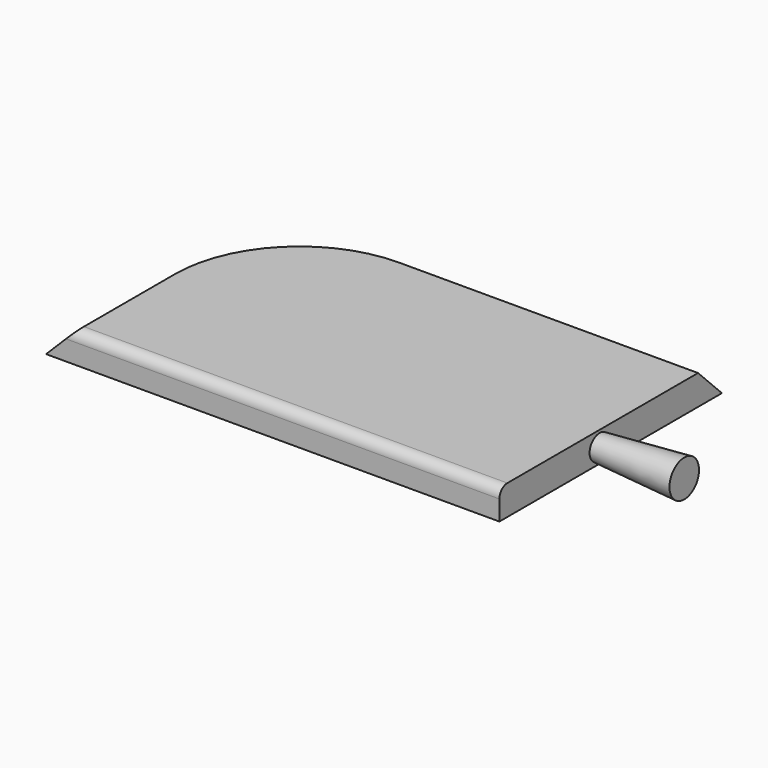
from build123d import *

# Parameters (mm, degrees)
F1_DEPTH    = 15.24
F2_T1_DEPTH = 217.8918149653
F2_T3_DEPTH = 128.5071697417
F2_T6_ANGLE = 90
F3_R        = 5.08
F4_R        = 6.3991299939
F5_DEPTH    = 43.18
F5_TAPER    = -4


# Not quite as in the source:
# - a fillet or chamfer that OpenCascade refuses, or shapes differently, is made with other operations: its cross-section is extruded or revolved along the edge and cut away or added


with BuildPart() as f1:
    # F0 (on Top) → F1 (new body)
    with BuildSketch(Plane.XY):
        with BuildLine():
            Line((120.7355335355, 76.0432109237), (-31.8355335355, 76.0432109237))
            ThreePointArc((-31.8355335355, 76.0432109237), (-94.697326383, 50.0050037712), (-120.7355335355, -12.8567890763))
            Line((-120.7355335355, -12.8567890763), (-120.7355335355, -76.0432109237))
            Line((-120.7355335355, -76.0432109237), (120.7355335355, -76.0432109237))
            Line((120.7355335355, -76.0432109237), (120.7355335355, 76.0432109237))
        make_face()
    extrude(amount=F1_DEPTH)

    # F2: chamfer of 25.4 on 1 edges, made by hand

    # F2_s2 → F2_t1 (cut)
    with BuildSketch(Plane.YZ.offset(-31.8355335355)):
        Polygon((76.0432109237, -10.16), (50.6432109237, 15.24), (76.0432109237, 15.24), align=None)
    extrude(amount=F2_T1_DEPTH, mode=Mode.SUBTRACT)

    # F2_s4 → F2_t3 (cut)
    with BuildSketch(Plane.XZ.offset(12.8567890763)):
        Polygon((-120.7355335355, -10.16), (-95.3355335355, 15.24), (-120.7355335355, 15.24), align=None)
    extrude(amount=F2_T3_DEPTH, mode=Mode.SUBTRACT)

    # F2_s5 → F2_t6 (revolve, cut)
    with BuildSketch(Plane.YZ.offset(-31.8355335355)):
        Polygon((76.0432109237, -10.16), (50.6432109237, 15.24), (76.0432109237, 15.24), align=None)
    revolve(axis=Axis((-31.8355335355, -12.8567890763, 15.24), (0, 0, 1)), revolution_arc=F2_T6_ANGLE, mode=Mode.SUBTRACT)

    # F3
    f3_edges = [f1.edges().sort_by_distance(p)[0] for p in [
        (12.7, -76.043211, 15.24),
    ]]
    fillet(f3_edges, radius=F3_R)

    # F4 (on face) → F5 (join)
    with BuildSketch(Plane.YZ.offset(120.7355335355)):
        with Locations((-12.1188843623, 7.419291418)):
            Circle(F4_R)
    extrude(amount=F5_DEPTH, taper=F5_TAPER)


solid = f1.part
